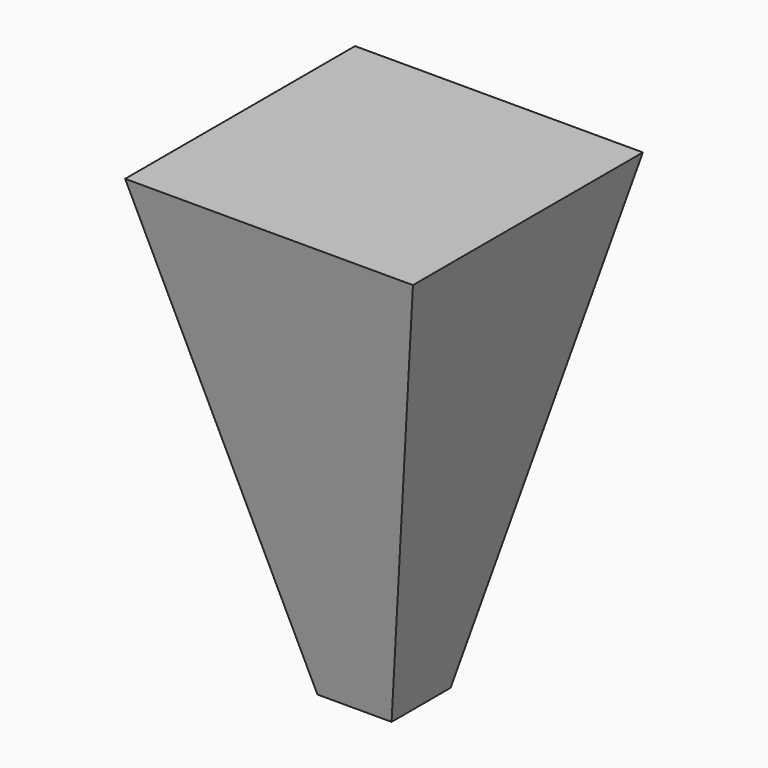
from build123d import *

# Parameters (mm, degrees)
F0_W                   = 383.1095849226
F0_H                   = 381
F1_DEPTH               = 75.438
F2_R                   = 5.08
F3_DEPTH               = 2390.14
DRAFT_F3_DRAFTED_ANGLE = -13


# Not quite as in the source:
# - an extrude with a draft is written as a straight extrude whose walls are then drafted


with BuildPart() as f1:
    # F0 (on Top) → F1 (new body)
    with BuildSketch(Plane.XY):
        with Locations((0.3764256835, -0.4907026887)):
            Rectangle(F0_W, F0_H)
    extrude(amount=F1_DEPTH)

    # F2
    f2_edges = [f1.edges().sort_by_distance(p)[0] for p in [
        (191.931218, -190.990703, 37.719),
        (-191.178367, -190.990703, 37.719),
        (191.931218, 190.009297, 37.719),
        (191.931218, -0.490703, 75.438),
        (0.376426, 190.009297, 75.438),
        (-191.178367, -0.490703, 75.438),
        (0.376426, -190.990703, 75.438),
        (-191.178367, 190.009297, 37.719),
    ]]
    fillet(f2_edges, radius=F2_R)


with BuildPart() as f3_drafted:
    # F0 (on Top) + F1_face (on face) → F3 (new body)
    with BuildSketch(Plane.XY):
        with Locations((0.3764256835, -0.4907026887)):
            Rectangle(F0_W, F0_H)
    with BuildSketch(Plane(origin=(0.3764256835, -0.4907026887, 0), x_dir=(1, 0, 0), z_dir=(0, 0, -1))):
        with BuildLine():
            Line((191.5547924613, -185.42), (191.5547924613, 185.42))
            ThreePointArc((191.5547924613, 185.42), (190.0668949097, 189.0121024484), (186.4747924613, 190.5))
            Line((186.4747924613, 190.5), (-186.4747924613, 190.5))
            ThreePointArc((-186.4747924613, 190.5), (-190.0668949097, 189.0121024484), (-191.5547924613, 185.42))
            Line((-191.5547924613, 185.42), (-191.5547924613, -185.42))
            ThreePointArc((-191.5547924613, -185.42), (-190.0668949097, -189.0121024484), (-186.4747924613, -190.5))
            Line((-186.4747924613, -190.5), (186.4747924613, -190.5))
            ThreePointArc((186.4747924613, -190.5), (190.0668949097, -189.0121024484), (191.5547924613, -185.42))
        make_face()
    extrude(amount=F3_DEPTH, dir=(0, 0, 1))

    # draft_F3_drafted
    draft_f3_drafted_walls = [f3_drafted.faces().sort_by_distance(p)[0] for p in [
        (191.9312181448, -0.4907026887, 1593.4266666667),
        (0.3764256835, 190.0092973113, 1593.4266666667),
        (-191.1783667778, -0.4907026887, 1593.4266666667),
        (0.3764256835, -190.9907026887, 1593.4266666667),
    ]]
    draft(draft_f3_drafted_walls, neutral_plane=Plane.XY, angle=DRAFT_F3_DRAFTED_ANGLE)


with BuildPart() as f1_1:
    add(f1.part)

    # join_F3_drafted: union F3_drafted
    add(f3_drafted.part)


solid = f1_1.part
